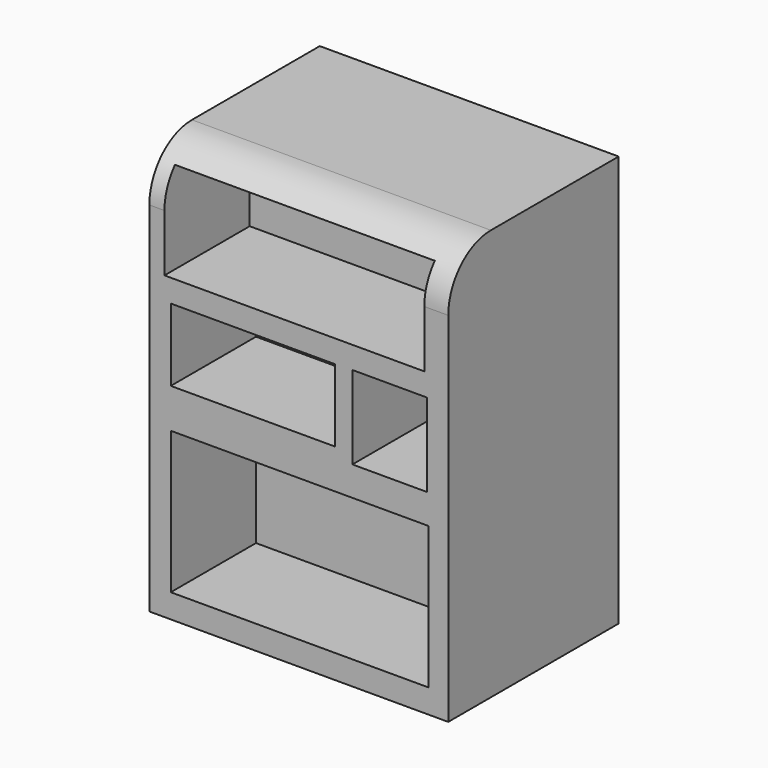
from build123d import *

# Parameters (mm, degrees)
F0_W        = 71.2871104479
F0_H        = 49.0286853164
F0_W_2      = 58.531470614
F0_H_2      = 36.0211754636
F0_W_3      = 60.9135755652
F0_H_3      = 33.0608540971
F1_DEPTH    = 50.8
F2_W        = 39.112127386
F2_H        = 17.2953940928
F2_W_2      = 17.7711145952
F2_H_2      = 19.8306103703
F2_W_3      = 61.416560784
F2_H_3      = 33.9031042531
F2_W_4      = 61.9626361877
F2_H_4      = 21.9576358795
F3_DEPTH    = 25.4
F4_T1_DEPTH = 134.7871104479


# Not quite as in the source:
# - a fillet or chamfer that OpenCascade refuses, or shapes differently, is made with other operations: its cross-section is extruded or revolved along the edge and cut away or added


with BuildPart() as f1:
    # F0 (on Front) → F1 (new body)
    with BuildSketch(Plane.XZ):
        with Locations((0, 24.5143426582)):
            Rectangle(F0_W, F0_H)
        with Locations((-0.6145685997, 23.0905877318)):
            Rectangle(F0_W_2, F0_H_2, mode=Mode.SUBTRACT)
        with Locations((0, -24.5143426582)):
            Rectangle(F0_W, F0_H)
        with Locations((0.2925068763, -25.7660689676)):
            Rectangle(F0_W_3, F0_H_3, mode=Mode.SUBTRACT)
        with Locations((-0.6145685997, 23.0905877318)):
            Rectangle(F0_W_2, F0_H_2)
        with Locations((0.2925068763, -25.7660689676)):
            Rectangle(F0_W_3, F0_H_3)
    extrude(amount=F1_DEPTH)

    # F2 (on face) → F3 (cut)
    with BuildSketch(Plane.XZ.offset(50.8)):
        with Locations((-10.9740667976, 8.6476970464)):
            Rectangle(F2_W, F2_H)
        with Locations((21.669532638, 7.5109825702)):
            Rectangle(F2_W_2, F2_H_2)
        with Locations((0.1781499013, -26.3703963719)):
            Rectangle(F2_W_3, F2_H_3)
        with Locations((-1.0527623817, 33.6884222925)):
            Rectangle(F2_W_4, F2_H_4)
    extrude(amount=-F3_DEPTH, mode=Mode.SUBTRACT)

    # F4: fillet of radius 12.7 on 1 edges, made by hand

    # F4_s2 → F4_t1 (cut)
    with BuildSketch(Plane.YZ.offset(-67.3935552239)):
        with BuildLine():
            ThreePointArc((-50.8, 36.3286853164), (-47.0802561211, 45.3089414375), (-38.1, 49.0286853164))
            Line((-38.1, 49.0286853164), (-50.8, 49.0286853164))
            Line((-50.8, 49.0286853164), (-50.8, 36.3286853164))
        make_face()
    extrude(amount=F4_T1_DEPTH, mode=Mode.SUBTRACT)


solid = f1.part
